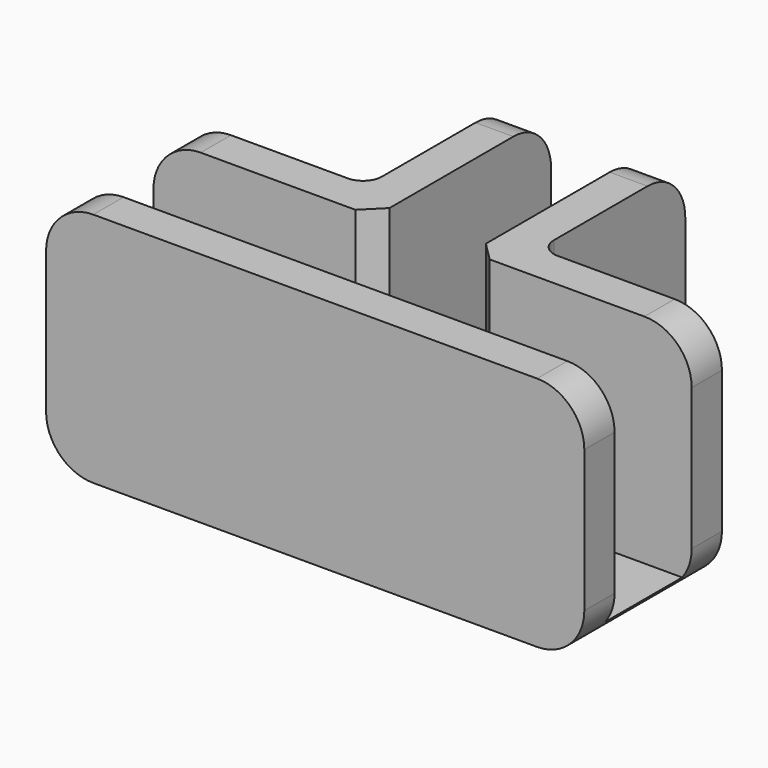
from build123d import *

# Parameters (mm, degrees)
F1_DEPTH       = 2
F2_DEPTH       = 25
F3_R           = 2
F4_T1_DEPTH    = 29
F4_T3_DEPTH    = 29
F4_T5_DEPTH    = 29
F4_T7_DEPTH    = 29
F4_T9_DEPTH    = 43.2
F4_T11_DEPTH   = 43.2
F5_R           = 2
F6_SIZE        = 2
F8_D           = 3.3
F8_CSINK_D     = 6
F8_CSINK_ANGLE = 90


# Not quite as in the source:
# - a fillet or chamfer that OpenCascade refuses, or shapes differently, is made with other operations: its cross-section is extruded or revolved along the edge and cut away or added


with BuildPart() as f1:
    # F0 (on Top) → F1 (new body)
    with BuildSketch(Plane.XY):
        Polygon((-28.4735770881, 0), (0, 0), (28.4735770881, 0), (28.4735770881, 10.2), (5.1, 10.2), (5.1, 33.5735770881), (-5.1, 33.5735770881), (-5.1, 10.2), (-28.4735770881, 10.2), align=None)
        Polygon((28.4735770881, 0), (0, 0), (-28.4735770881, 0), (-28.4735770881, -4), (0, -4), (28.4735770881, -4), align=None)
        Polygon((5.1, 10.2), (28.4735770881, 10.2), (28.4735770881, 14.2), (9.1, 14.2), (9.1, 33.5735770881), (5.1, 33.5735770881), align=None)
        Polygon((-28.4735770881, 14.2), (-28.4735770881, 10.2), (-5.1, 10.2), (-5.1, 33.5735770881), (-9.1, 33.5735770881), (-9.1, 14.2), align=None)
    extrude(amount=F1_DEPTH)

    # F0 (on Top) → F2 (join)
    with BuildSketch(Plane.XY):
        Polygon((-28.4735770881, 14.2), (-28.4735770881, 10.2), (-5.1, 10.2), (-5.1, 33.5735770881), (-9.1, 33.5735770881), (-9.1, 14.2), align=None)
        Polygon((5.1, 10.2), (28.4735770881, 10.2), (28.4735770881, 14.2), (9.1, 14.2), (9.1, 33.5735770881), (5.1, 33.5735770881), align=None)
        Polygon((28.4735770881, 0), (0, 0), (-28.4735770881, 0), (-28.4735770881, -4), (0, -4), (28.4735770881, -4), align=None)
    extrude(amount=F2_DEPTH)

    # F3
    f3_edges = [f1.edges().sort_by_distance(p)[0] for p in [
        (9.1, 14.2, 12.5),
    ]]
    fillet(f3_edges, radius=F3_R)

    # F4: fillet of radius 5 on 9 edges, made by hand

    # F4_s2 → F4_t1 (cut)
    with BuildSketch(Plane.XZ.offset(-12.5)):
        with BuildLine():
            ThreePointArc((28.4735770881, 20), (27.0091109941, 23.5355339059), (23.4735770881, 25))
            Line((23.4735770881, 25), (28.4735770881, 25))
            Line((28.4735770881, 25), (28.4735770881, 20))
        make_face()
        with BuildLine():
            ThreePointArc((-28.4735770881, 20), (-27.0091109941, 23.5355339059), (-23.4735770881, 25))
            Line((-23.4735770881, 25), (-28.4735770881, 25))
            Line((-28.4735770881, 25), (-28.4735770881, 20))
        make_face()
    extrude(amount=F4_T1_DEPTH, mode=Mode.SUBTRACT)

    # F4_s4 → F4_t3 (cut)
    with BuildSketch(Plane.XZ.offset(-26.7)):
        with BuildLine():
            ThreePointArc((28.4735770881, 20), (27.0091109941, 23.5355339059), (23.4735770881, 25))
            Line((23.4735770881, 25), (28.4735770881, 25))
            Line((28.4735770881, 25), (28.4735770881, 20))
        make_face()
        with BuildLine():
            ThreePointArc((-28.4735770881, 20), (-27.0091109941, 23.5355339059), (-23.4735770881, 25))
            Line((-23.4735770881, 25), (-28.4735770881, 25))
            Line((-28.4735770881, 25), (-28.4735770881, 20))
        make_face()
    extrude(amount=F4_T3_DEPTH, mode=Mode.SUBTRACT)

    # F4_s6 → F4_t5 (cut)
    with BuildSketch(Plane.YZ.offset(-21.6)):
        with BuildLine():
            ThreePointArc((33.5735770881, 20), (32.1091109941, 23.5355339059), (28.5735770881, 25))
            Line((28.5735770881, 25), (33.5735770881, 25))
            Line((33.5735770881, 25), (33.5735770881, 20))
        make_face()
    extrude(amount=F4_T5_DEPTH, mode=Mode.SUBTRACT)

    # F4_s8 → F4_t7 (cut)
    with BuildSketch(Plane.YZ.offset(-7.4)):
        with BuildLine():
            ThreePointArc((33.5735770881, 20), (32.1091109941, 23.5355339059), (28.5735770881, 25))
            Line((28.5735770881, 25), (33.5735770881, 25))
            Line((33.5735770881, 25), (33.5735770881, 20))
        make_face()
    extrude(amount=F4_T7_DEPTH, mode=Mode.SUBTRACT)

    # F4_s10 → F4_t9 (cut)
    with BuildSketch(Plane.XZ.offset(-26.7)):
        with BuildLine():
            ThreePointArc((-23.4735770881, 0), (-27.0091109941, 1.4644660941), (-28.4735770881, 5))
            Line((-28.4735770881, 5), (-28.4735770881, 0))
            Line((-28.4735770881, 0), (-23.4735770881, 0))
        make_face()
        with BuildLine():
            ThreePointArc((23.4735770881, 0), (27.0091109941, 1.4644660941), (28.4735770881, 5))
            Line((28.4735770881, 5), (28.4735770881, 0))
            Line((28.4735770881, 0), (23.4735770881, 0))
        make_face()
    extrude(amount=F4_T9_DEPTH, mode=Mode.SUBTRACT)

    # F4_s12 → F4_t11 (cut)
    with BuildSketch(Plane.YZ.offset(-21.6)):
        with BuildLine():
            ThreePointArc((28.5735770881, 0), (32.1091109941, 1.4644660941), (33.5735770881, 5))
            Line((33.5735770881, 5), (33.5735770881, 0))
            Line((33.5735770881, 0), (28.5735770881, 0))
        make_face()
    extrude(amount=F4_T11_DEPTH, mode=Mode.SUBTRACT)

    # F5
    f5_edges = [f1.edges().sort_by_distance(p)[0] for p in [
        (-9.1, 14.2, 12.5),
    ]]
    fillet(f5_edges, radius=F5_R)

    # F6
    f6_edges = [f1.edges().sort_by_distance(p)[0] for p in [
        (5.1, 10.2, 13.5),
        (-5.1, 10.2, 13.5),
    ]]
    chamfer(f6_edges, length=F6_SIZE)

    # F8 (through all)
    with Locations(Plane(origin=(0, 0, 0), x_dir=(1, 0, 0), z_dir=(0, 0, -1))):
        with Locations((-15, -5.1), (0, -20.1), (15, -5.1)):
            CounterSinkHole(F8_D / 2, F8_CSINK_D / 2, counter_sink_angle=F8_CSINK_ANGLE)


solid = f1.part
